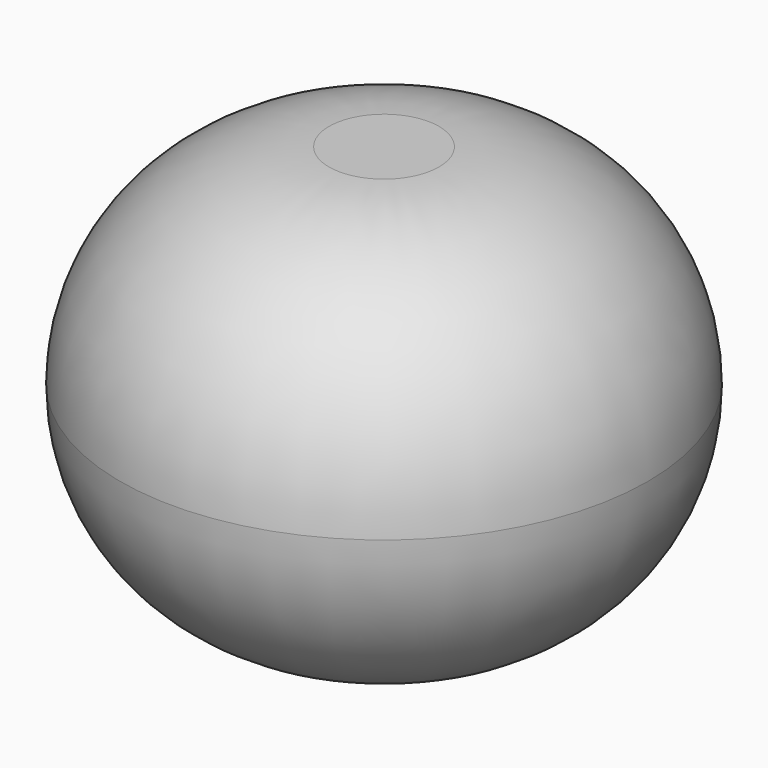
from build123d import *

# Parameters (mm, degrees)
F0_R     = 64.1724242316
F1_DEPTH = 101.6
F2_R     = 50.79999


# Not quite as in the source:
# - a fillet or chamfer is up to 0.001 mm smaller than in the source, because OpenCascade refuses the exact size


with BuildPart() as f1:
    # F0 (on Top) → F1 (new body)
    with BuildSketch(Plane.XY):
        Circle(F0_R)
    extrude(amount=F1_DEPTH)

    # F2 (radius 50.8 in the source; OpenCascade refuses exactly that, so slightly less here)
    f2_edges = [f1.edges().sort_by_distance(p)[0] for p in [
        (-64.172424, 0, 101.6),
        (-64.172424, 0, 0),
    ]]
    fillet(f2_edges, radius=F2_R)


solid = f1.part
